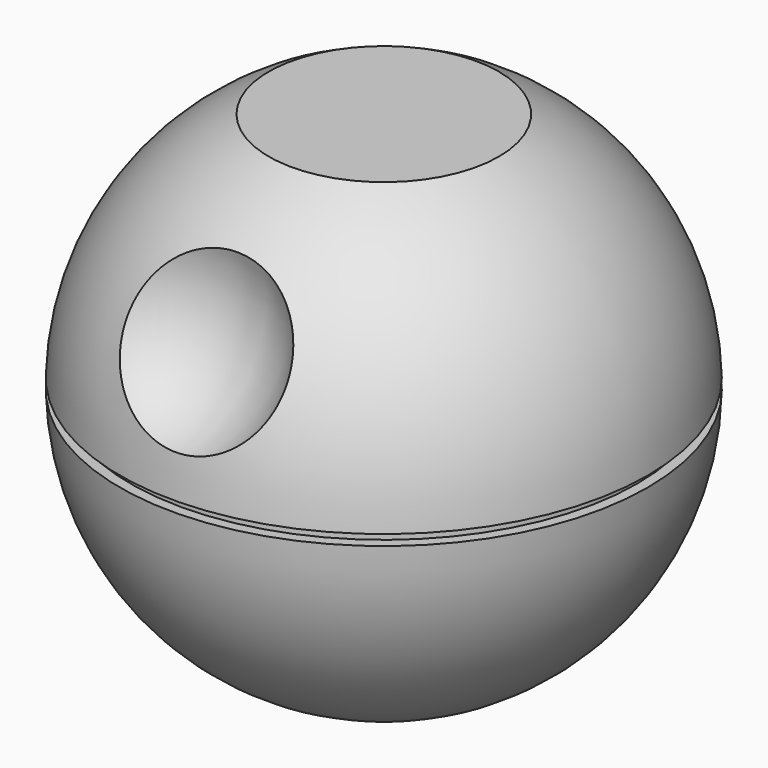
from build123d import *

# Parameters (mm, degrees)
F4_W          = 126.554620702
F4_H          = 16.890758596
F5_DEPTH      = 25
F5_DEPTH_BACK = 25
F6_W          = 22.8272504394
F6_H          = 2


# Not quite as in the source:
# - a pattern or mirror of a feature is missing from the dataset's text; its kind, count and spacing are read off the source's solid


with BuildPart() as f1:
    # F0 (on Front) → F1 (revolve)
    with BuildSketch(Plane.XZ):
        with BuildLine():
            Line((0, 50), (0, -50))
            ThreePointArc((0, -50), (50, 0), (0, 50))
        make_face()
    revolve(axis=Axis((0, 0, 0), (0, 0, -1)))

    # F2 (on Right) → F3 (revolve, cut)
    with BuildSketch(Plane.YZ):
        with BuildLine():
            Line((-55, 52.4620511452), (-56.5292847679, 7.5011055772))
            ThreePointArc((-56.5292847679, 7.5011055772), (-33.8192423865, 29.2351357427), (-55, 52.4620511452))
        make_face()
    revolve(axis=Axis((0, -55.7646423839, 29.9815783612), (0, -0.033993967, -0.9994220381)), mode=Mode.SUBTRACT)

    # F4 (on Front) → F5 (cut, two sides)
    with BuildSketch(Plane.XZ) as f5_sk:
        with Locations((-0.5138665438, 53.445379298)):
            Rectangle(F4_W, F4_H)
    f5 = extrude(amount=-F5_DEPTH, mode=Mode.SUBTRACT) + extrude(f5_sk.sketch, amount=F5_DEPTH_BACK, mode=Mode.SUBTRACT)

    # F5_copies: F5 across plane
    add(f5.mirror(Plane(origin=(0, 0, 0), x_dir=(-1, 0, 0), z_dir=(0, 0, -1))), mode=Mode.SUBTRACT)

    # F6 (on Front) → F7 (revolve, cut)
    with BuildSketch(Plane.XZ):
        with Locations((-59.4136252197, 0)):
            Rectangle(F6_W, F6_H)
    revolve(axis=Axis((0, 0, 0), (0, 0, -1)), mode=Mode.SUBTRACT)


solid = f1.part
